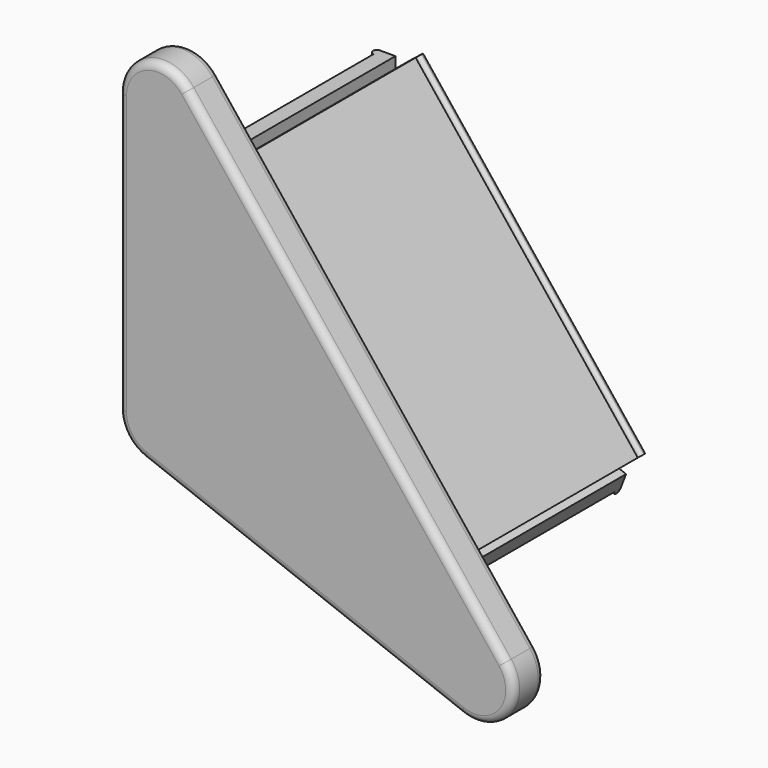
from build123d import *

# Parameters (mm, degrees)
F0_W      = 2.54
F0_H      = 29.1471965611
F1_DEPTH  = 6.35
F2_DEPTH  = 39.37
F3_W      = 1.27
F3_H      = 58.7419511778
F4_DEPTH  = 0.635
F5_R      = 0.63499
F6_W      = 38.6529213808
F6_H      = 1.27
F7_DEPTH  = 0.635
F8_R      = 0.63499
F9_W      = 1.27
F9_H      = 29.1471965611
F10_DEPTH = 0.635
F11_R     = 0.63499
F12_R     = 1.27


# Not quite as in the source:
# - a fillet or chamfer is up to 0.001 mm smaller than in the source, because OpenCascade refuses the exact size


with BuildPart() as f1:
    # F0 (on Front) → F1 (new body)
    with BuildSketch(Plane.XZ):
        with BuildLine():
            Line((57.1427482982, -61.7985644783), (4.9742740829, 3.9470365205))
            ThreePointArc((4.9742740829, 3.9470365205), (-2.0899592777, 5.9962129759), (-6.3499999957, -1.22e-08))
            Line((-6.3499999957, -1.22e-08), (-6.3499999957, -45.7199999971))
            ThreePointArc((-6.3499999957, -45.7199999971), (-5.2332012935, -49.3166796015), (-2.2756364753, -51.6482357053))
            Line((-2.2756364754, -51.6482357053), (49.89283774, -71.6738367193))
            ThreePointArc((49.89283774, -71.6738367193), (57.2871568315, -69.5034711949), (57.1427482982, -61.7985644783))
        make_face()
        Polygon((0, -10.3762075305), (0, 0), (6.8810137765, -8.6718347243), (43.39386847, -54.6873567827), (52.1684742327, -65.7456010206), (39.5421703506, -60.8988170648), (3.4565595225, -47.0468488857), (0, -45.72), (0, -39.5234040916), align=None, mode=Mode.SUBTRACT)
        Polygon((6.8810137765, -8.6718347243), (0, 0), (0, -10.3762075305), (2.54, -10.3762075305), (2.54, -39.5234040916), (0, -39.5234040916), (0, -45.72), (3.4565595225, -47.0468488857), (4.3668141144, -44.6755546023), (40.4524249424, -58.5275227815), (39.5421703506, -60.8988170648), (52.1684742327, -65.7456010206), (43.39386847, -54.6873567827), (41.4041588386, -56.2661713958), (4.891304145, -10.2506493374), align=None)
        with Locations((1.27, -24.949805811)):
            Rectangle(F0_W, F0_H)
        Polygon((43.39386847, -54.6873567827), (6.8810137765, -8.6718347243), (4.891304145, -10.2506493374), (41.4041588386, -56.2661713958), align=None)
        Polygon((4.3668141144, -44.6755546023), (3.4565595225, -47.0468488857), (39.5421703506, -60.8988170648), (40.4524249424, -58.5275227815), align=None)
    extrude(amount=F1_DEPTH)

    # F12
    f12_edges = [f1.edges().sort_by_distance(p)[0] for p in [
        (-6.35, -6.35, -22.86),
        (-6.35, 0, -22.86),
    ]]
    fillet(f12_edges, radius=F12_R)


with BuildPart() as f2:
    # F0 (on Front) → F2 (new body)
    with BuildSketch(Plane.XZ):
        with Locations((1.27, -24.949805811)):
            Rectangle(F0_W, F0_H)
    extrude(amount=-F2_DEPTH)

    # F9 (on face) → F10 (join)
    with BuildSketch(Plane(origin=(0, 0, 0), x_dir=(0, -1, 0), z_dir=(-1, 0, 0))):
        with Locations((-38.735, -24.949805811)):
            Rectangle(F9_W, F9_H)
    extrude(amount=F10_DEPTH)

    # F11 (radius 0.635 in the source; OpenCascade refuses exactly that, so slightly less here)
    f11_edges = [f2.edges().sort_by_distance(p)[0] for p in [
        (-0.635, 38.1, -24.949806),
        (-0.635, 39.37, -24.949806),
    ]]
    fillet(f11_edges, radius=F11_R)


with BuildPart() as f2b:
    # F0 (on Front) → F2, piece 2 (new body)
    with BuildSketch(Plane.XZ):
        Polygon((4.3668141144, -44.6755546023), (3.4565595225, -47.0468488857), (39.5421703506, -60.8988170648), (40.4524249424, -58.5275227815), align=None)
    extrude(amount=-F2_DEPTH)

    # F6 (on face) → F7 (join)
    with BuildSketch(Plane(origin=(-15.2963256614, 0, -39.8482907104), x_dir=(0.9335804265, 0, -0.3583679495), z_dir=(-0.3583679495, 0, -0.9335804265))):
        with Locations((39.4135197714, -38.735)):
            Rectangle(F6_W, F6_H)
    extrude(amount=F7_DEPTH)

    # F8 (radius 0.635 in the source; OpenCascade refuses exactly that, so slightly less here)
    f8_edges = [f2b.edges().sort_by_distance(p)[0] for p in [
        (21.271801, 38.1, -54.565657),
        (21.271801, 39.37, -54.565657),
    ]]
    fillet(f8_edges, radius=F8_R)


with BuildPart() as f2c:
    # F0 (on Front) → F2, piece 3 (new body)
    with BuildSketch(Plane.XZ):
        Polygon((43.39386847, -54.6873567827), (6.8810137765, -8.6718347243), (4.891304145, -10.2506493374), (41.4041588386, -56.2661713958), align=None)
    extrude(amount=-F2_DEPTH)

    # F3 (on face) → F4 (join)
    with BuildSketch(Plane(origin=(0, 0, 0), x_dir=(0, 1, 0), z_dir=(0.7833502486, 0, 0.6215805563))):
        with Locations((38.735, -40.4411638473)):
            Rectangle(F3_W, F3_H)
    extrude(amount=F4_DEPTH)

    # F5 (radius 0.635 in the source; OpenCascade refuses exactly that, so slightly less here)
    f5_edges = [f2c.edges().sort_by_distance(p)[0] for p in [
        (25.634869, 38.1, -31.284892),
        (25.634869, 39.37, -31.284892),
    ]]
    fillet(f5_edges, radius=F5_R)


solid = Compound([f1.part, f2.part, f2b.part, f2c.part])
